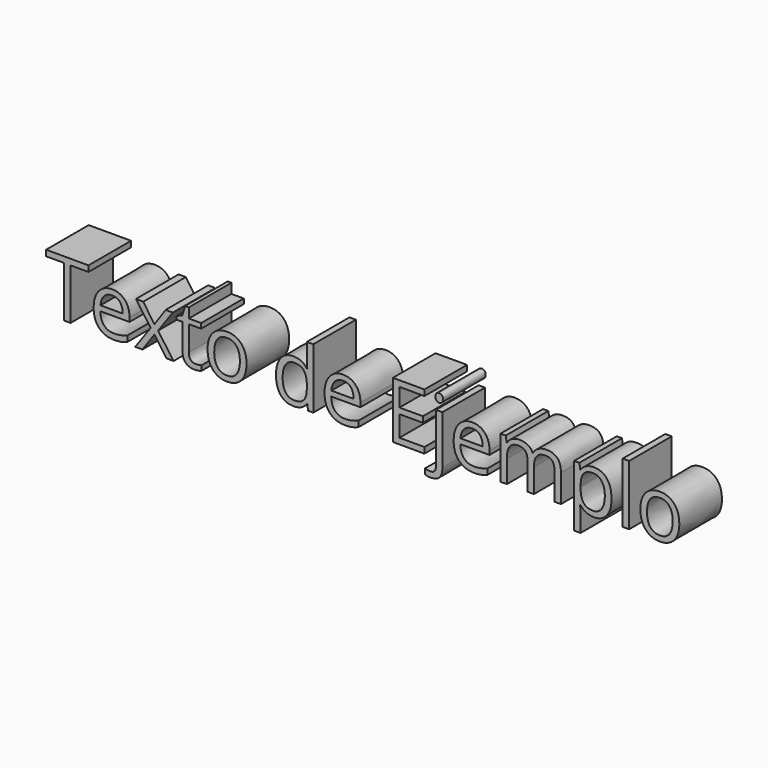
from build123d import *

# Parameters (mm, degrees)
F0_TEXT_SIZE = 18.890244611
F1_DEPTH     = 12.7


# Not quite as in the source:
# - Text() gives the source's letters only with a copy of the font that has no kerning and outlines rounded to 1/6400 em; it was checked with that copy


with BuildPart() as f1:
    # F0 (on Front) → F1 (new body)
    with BuildSketch(Plane.XZ):
        with Locations((-76.2, -4.3625770381)):
            Text('Texto de Ejemplo', F0_TEXT_SIZE, font='Open Sans', text_align=(TextAlign.LEFT, TextAlign.BOTTOM))
    extrude(amount=F1_DEPTH)


solid = f1.part
